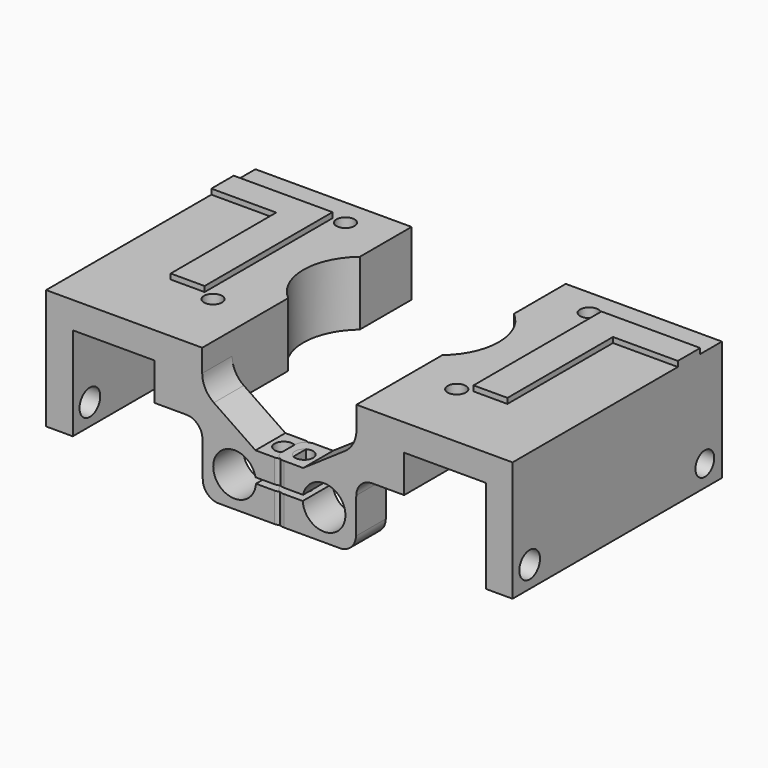
from build123d import *

# Parameters (mm, degrees)
F1_DEPTH      = 7
F2_DEPTH      = 42
F3_R          = 1.7
F3_R_2        = 11
F4_DEPTH      = 12.001
F5_R          = 4
F6_DEPTH      = 10
F7_DEPTH      = 12.001
F8_R          = 1.4
F9_DEPTH      = 10.9920075553
F8_R_2        = 1.7
F10_DEPTH     = 4.4348209087
F11_R         = 5
F12_R         = 3
F13_R         = 3
F14_R         = 2
F15_R         = 2.2
F15_R_2       = 2.4255023423
F16_DEPTH     = 6
F17_TEXT_SIZE = 41.9437823343
F18_DEPTH     = 1


# Not quite as in the source:
# - a feature names something its author has since deleted; it is built from what else it names
# - Text() gives the source's letters only with a copy of the font that has no kerning and outlines rounded to 1/6400 em; it was checked with that copy


with BuildPart() as f1:
    # F0 (on Front) → F1 (new body)
    with BuildSketch(Plane.XZ):
        Polygon((-18.6721007523, 29.8099789735), (-18.6721007523, 7.3259699669), (-13.6721007523, 7.3259699669), (-13.6721007523, 24.8099789735), (1.6278992477, 24.8099789735), (1.6278992477, 17.8099789735), (10.5637966118, 17.8099789735), (10.5637966118, 22.9406704692), (10.5637966118, 29.8099789735), align=None)
        Polygon((20.5301751077, 16.1394868046), (10.5637966118, 22.9406704692), (10.5637966118, 17.8099789735), (10.6940201178, 5.1484792493), (26.1186601057, 5.1484792493), (26.1186601057, 10.6682249423), (18.7860510706, 10.6682249423), (18.7860510706, 11.7046658959), (26.0896428882, 11.7046658959), (26.0896428882, 16.1394868046), align=None)
    extrude(amount=F1_DEPTH)

    # F0 (on Front) → F2 (join)
    with BuildSketch(Plane.XZ):
        Polygon((-18.6721007523, 29.8099789735), (-18.6721007523, 7.3259699669), (-13.6721007523, 7.3259699669), (-13.6721007523, 24.8099789735), (1.6278992477, 24.8099789735), (1.6278992477, 17.8099789735), (10.5637966118, 17.8099789735), (10.5637966118, 22.9406704692), (10.5637966118, 29.8099789735), align=None)
    extrude(amount=-F2_DEPTH)

    # F3 (on face) → F4 (cut, through all)
    with BuildSketch(Plane(origin=(0, 0, 17.8099789735), x_dir=(1, 0, 0), z_dir=(0, 0, -1))):
        with Locations((2.1850741468, -6)):
            Circle(F3_R)
        with Locations((2.1850741468, -37)):
            Circle(F3_R)
        with Locations((17.6850741468, -21.5)):
            Circle(F3_R_2)
    extrude(amount=-F4_DEPTH, mode=Mode.SUBTRACT)

    # F5 (on face) → F6 (cut)
    with BuildSketch(Plane.XZ.offset(7)):
        with Locations((16.6278992477, 10.8989789735)):
            Circle(F5_R)
    extrude(amount=-F6_DEPTH, mode=Mode.SUBTRACT)

    # F3 (on face) → F7 (cut, through all)
    with BuildSketch(Plane(origin=(0, 0, 17.8099789735), x_dir=(1, 0, 0), z_dir=(0, 0, -1))):
        with Locations((2.1850741468, -6)):
            Circle(F3_R)
        with Locations((2.1850741468, -37)):
            Circle(F3_R)
        with Locations((17.6850741468, -21.5)):
            Circle(F3_R_2)
    extrude(amount=-F7_DEPTH, mode=Mode.SUBTRACT)

    # F8 (on face) → F9 (cut, through all)
    with BuildSketch(Plane.XY.offset(16.1394868046)):
        with Locations((23.0896428882, -3.5767070949)):
            Circle(F8_R)
    extrude(amount=-F9_DEPTH, mode=Mode.SUBTRACT)

    # F8 (on face) → F10 (cut, through all)
    with BuildSketch(Plane.XY.offset(16.1394868046)):
        with Locations((23.0896428882, -3.5767070949)):
            Circle(F8_R_2)
        with Locations((23.0896428882, -3.5767070949)):
            Circle(F8_R, mode=Mode.SUBTRACT)
    extrude(amount=-F10_DEPTH, mode=Mode.SUBTRACT)

    # F11
    f11_edges = [f1.edges().sort_by_distance(p)[0] for p in [
        (10.563797, -3.5, 22.94067),
    ]]
    fillet(f11_edges, radius=F11_R)

    # F12
    f12_edges = [f1.edges().sort_by_distance(p)[0] for p in [
        (10.563797, -3.5, 17.809979),
    ]]
    fillet(f12_edges, radius=F12_R)

    # F13
    f13_edges = [f1.edges().sort_by_distance(p)[0] for p in [
        (10.69402, -3.5, 5.148479),
    ]]
    fillet(f13_edges, radius=F13_R)

    # F14
    f14_edges = [f1.edges().sort_by_distance(p)[0] for p in [
        (26.089643, -7, 13.922076),
        (26.11866, -7, 7.908352),
        (26.089643, 0, 13.922076),
        (26.11866, 0, 7.908352),
    ]]
    fillet(f14_edges, radius=F14_R)

    # F15 (on face) → F16 (cut)
    with BuildSketch(Plane(origin=(-18.6721007523, 0, 0), x_dir=(0, -1, 0), z_dir=(-1, 0, 0))):
        with Locations((-38, 11.3259699669)):
            Circle(F15_R)
        with Locations((3, 11.3259699669)):
            Circle(F15_R_2)
    extrude(amount=-F16_DEPTH, mode=Mode.SUBTRACT)

    # F17 (on face) → F18 (join)
    with BuildSketch(Plane.XY.offset(29.8099789735)):
        with Locations(Location((3.5908724648, 36.9253193088), (0, 0, 180))):
            Text('L', F17_TEXT_SIZE, font='Open Sans', font_style=FontStyle.BOLD, text_align=(TextAlign.LEFT, TextAlign.BOTTOM))
    extrude(amount=F18_DEPTH)


with BuildPart() as f19_1:
    # F19: instance of F1
    add(f1.part.mirror(Plane.YZ))


with BuildPart() as f19_1_1:
    # F20: moved
    add(f19_1.part.moved(Location((50, 0, 0))))


solid = Compound([f1.part, f19_1_1.part])
